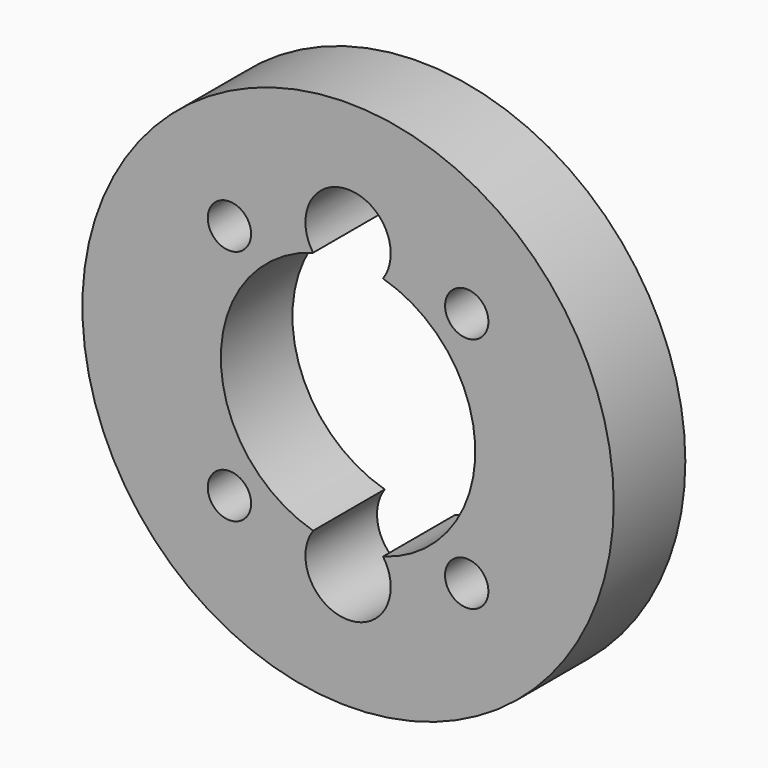
from build123d import *

# Parameters (mm, degrees)
F0_R            = 19
F1_DEPTH        = 6.4
F2_R            = 1.55
F3_DEPTH        = 25.4
F3_COPIES_COUNT = 4
F4_R            = 9.1
F5_DEPTH        = 6.401
F6_R            = 3.05
F7_DEPTH        = 6.401


# Not quite as in the source:
# - a pattern or mirror of a feature is missing from the dataset's text; its kind, count and spacing are read off the source's solid


with BuildPart() as f1:
    # F0 (on Front) → F1 (new body)
    with BuildSketch(Plane.XZ):
        Circle(F0_R)
    extrude(amount=F1_DEPTH)

    # F2 (on Front) → F3 (cut)
    with BuildSketch(Plane.XZ):
        with Locations((8.4852813742, 8.4852813742)):
            Circle(F2_R)
    f3 = extrude(amount=F3_DEPTH, mode=Mode.SUBTRACT)

    # F3_copies: F3 ×4 about axis
    f3_copies_axis = Axis((0, 0, 0), (0, 1, 0))
    for i in range(1, F3_COPIES_COUNT):
        add(f3.rotate(f3_copies_axis, i * 360 / F3_COPIES_COUNT), mode=Mode.SUBTRACT)

    # F4 (on Front) → F5 (cut, through all)
    with BuildSketch(Plane.XZ):
        Circle(F4_R)
    extrude(amount=F5_DEPTH, mode=Mode.SUBTRACT)

    # F6 (on Front) → F7 (cut, through all)
    with BuildSketch(Plane.XZ):
        with Locations((0, 10.5)):
            Circle(F6_R)
        with Locations((0, -10.5)):
            Circle(F6_R)
    extrude(amount=F7_DEPTH, mode=Mode.SUBTRACT)


solid = f1.part
